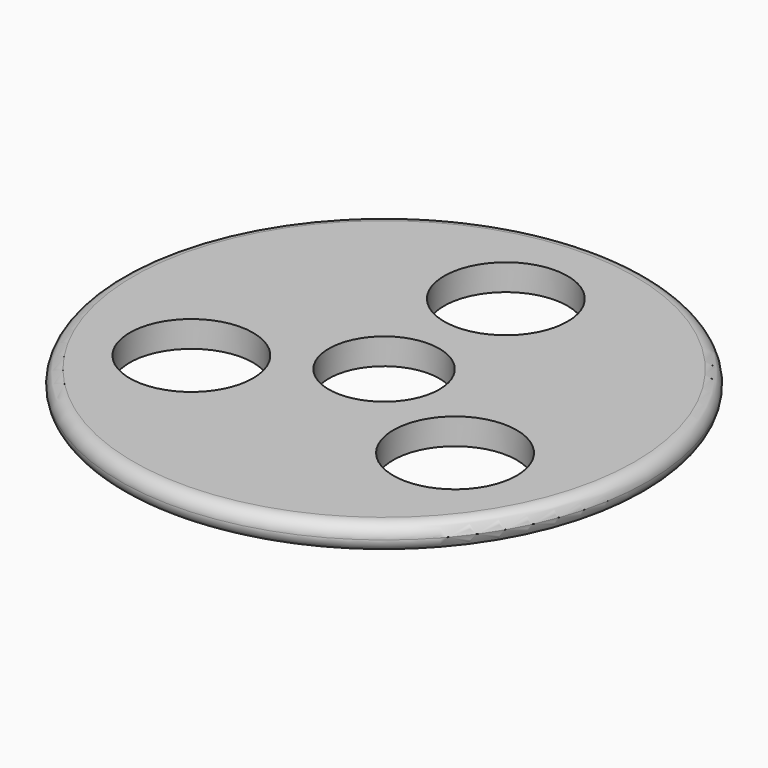
from build123d import *

# Parameters (mm, degrees)
F0_R     = 70.2853794577
F0_R_2   = 16.4264849476
F0_R_3   = 14.7171878195
F1_DEPTH = 7
F2_R     = 3.49999


# Not quite as in the source:
# - a fillet or chamfer is up to 0.001 mm smaller than in the source, because OpenCascade refuses the exact size


with BuildPart() as f1:
    # F0 (on Top) → F1 (new body)
    with BuildSketch(Plane.XY):
        Circle(F0_R)
        with Locations((-35.0998191676, -20.2648900449)):
            Circle(F0_R_2, mode=Mode.SUBTRACT)
        Circle(F0_R_3, mode=Mode.SUBTRACT)
        with Locations((35.0998191676, -20.2648900449)):
            Circle(F0_R_2, mode=Mode.SUBTRACT)
        with Locations((0, 40.5297800899)):
            Circle(F0_R_2, mode=Mode.SUBTRACT)
    extrude(amount=F1_DEPTH)

    # F2 (radius 3.5 in the source; OpenCascade refuses exactly that, so slightly less here)
    f2_edges = [f1.edges().sort_by_distance(p)[0] for p in [
        (-70.285379, 0, 7),
        (-70.285379, 0, 0),
    ]]
    fillet(f2_edges, radius=F2_R)


solid = f1.part
